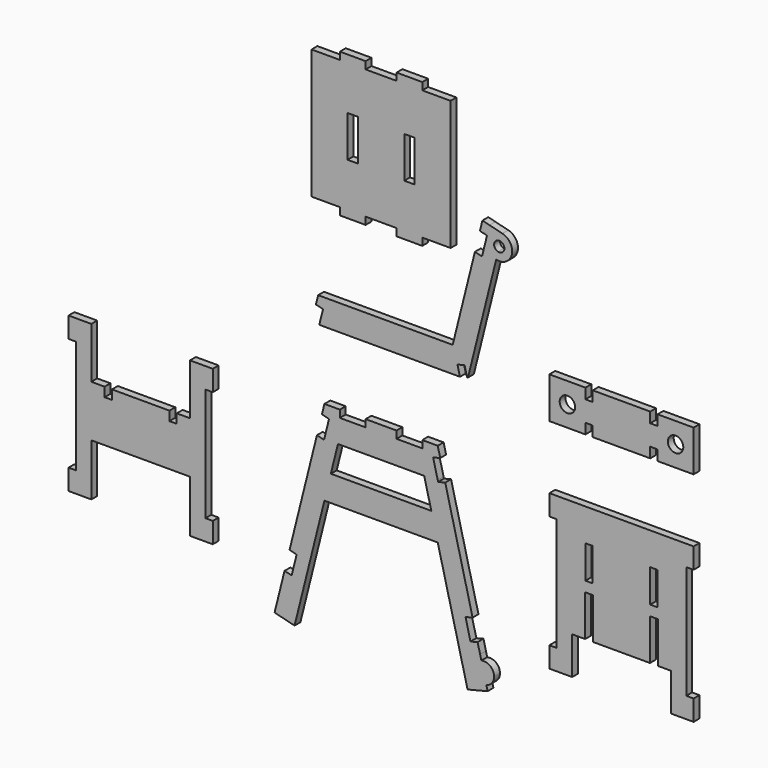
from build123d import *

# Parameters (mm, degrees)
F1_W     = 25.4
F1_H     = 101.6
F1_W_2   = 63.5
F1_H_2   = 18.034
F2_DEPTH = 18.034
F3_DEPTH = 18.034
F1_R     = 19.05
F4_DEPTH = 18.034
F1_W_3   = 18.034
F1_H_3   = 50.8
F1_H_4   = 25.4
F5_DEPTH = 18.034
F6_DEPTH = 18.034
F7_DEPTH = 18.034


# Not quite as in the source:
# - a variable given as a bare number and used for a length is read in inches; the dataset says mm whatever the document's units were


with BuildPart() as f2:
    # F1 (on Front) → F2 (new body)
    with BuildSketch(Plane.XZ):
        Polygon((91.1463229646, 1251.966), (91.1463229646, 932.434), (160.9963229646, 932.434), (224.4963229646, 932.434), (300.6963229646, 932.434), (364.1963229646, 932.434), (434.0463229646, 932.434), (434.0463229646, 1251.966), (364.1963229646, 1251.966), (300.6963229646, 1251.966), (224.4963229646, 1251.966), (160.9963229646, 1251.966), align=None)
        with Locations((192.7463229646, 1092.2)):
            Rectangle(F1_W, F1_H, mode=Mode.SUBTRACT)
        with Locations((332.4463229646, 1092.2)):
            Rectangle(F1_W, F1_H, mode=Mode.SUBTRACT)
        with Locations((332.4463229646, 1260.983)):
            Rectangle(F1_W_2, F1_H_2)
        with Locations((192.7463229646, 1260.983)):
            Rectangle(F1_W_2, F1_H_2)
        with Locations((192.7463229646, 923.417)):
            Rectangle(F1_W_2, F1_H_2)
        with Locations((332.4463229646, 923.417)):
            Rectangle(F1_W_2, F1_H_2)
    extrude(amount=F2_DEPTH)


with BuildPart() as f3:
    # F1 (on Front) → F3 (new body)
    with BuildSketch(Plane.XZ):
        with BuildLine():
            Line((143.9654091439, 723.9), (143.9654091439, 660.4))
            Line((143.9654091439, 660.4), (423.3654091439, 660.4))
            Line((423.3654091439, 660.4), (457.1344953232, 660.4))
            Line((457.1344953232, 660.4), (450.989679175, 685.0455114474))
            Line((450.989679175, 685.0455114474), (468.4879923026, 689.4083309127))
            Line((468.4879923026, 689.4083309127), (474.6328084508, 664.7628194652))
            Line((474.6328084508, 664.7628194652), (476.9525607092, 665.3411986629))
            Line((476.9525607092, 665.3411986629), (546.3859672195, 943.8233816452))
            ThreePointArc((546.3859672195, 943.8233816452), (523.2600980956, 982.3112911398), (561.7480075901, 1005.4371602637))
            Line((561.7480075901, 1005.4371602637), (529.955297823, 1013.363973095))
            Line((529.955297823, 1013.363973095), (523.8104816747, 988.7184616476))
            Line((523.8104816747, 988.7184616476), (511.5208493783, 939.4274387527))
            Line((511.5208493783, 939.4274387527), (494.0225362506, 943.790258218))
            Line((494.0225362506, 943.790258218), (439.1977373244, 723.9))
            Line((439.1977373244, 723.9), (423.3654091439, 723.9))
            Line((423.3654091439, 723.9), (143.9654091439, 723.9))
        make_face()
        Polygon((110.1963229646, 660.4), (143.9654091439, 660.4), (143.9654091439, 723.9), (107.4425649535, 723.9), (101.9152340593, 701.7310866364), (119.413547187, 697.3682671711), align=None)
        Polygon((512.4569846953, 1017.7267925602), (506.3121685471, 993.0812811128), (523.8104816747, 988.7184616476), (529.955297823, 1013.363973095), align=None)
        with BuildLine():
            ThreePointArc((561.7480075901, 1005.4371602637), (523.2600980956, 982.3112911398), (546.3859672195, 943.8233816452))
            Line((546.3859672195, 943.8233816452), (550.9945793307, 962.3075152308))
            ThreePointArc((550.9945793307, 962.3075152308), (541.7442316811, 977.7026790286), (557.139395479, 986.9530266782))
            Line((557.139395479, 986.9530266782), (561.7480075901, 1005.4371602637))
        make_face()
        with BuildLine():
            Line((550.9945793307, 962.3075152308), (546.3859672195, 943.8233816452))
            ThreePointArc((546.3859672195, 943.8233816452), (573.6142392464, 949.6109295275), (585.8169874048, 974.6302709545))
            ThreePointArc((585.8169874048, 974.6302709545), (579.0863288318, 994.1775227961), (561.7480075901, 1005.4371602637))
            Line((561.7480075901, 1005.4371602637), (557.139395479, 986.9530266782))
            ThreePointArc((557.139395479, 986.9530266782), (564.0747239756, 982.4491716911), (566.7669874048, 974.6302709545))
            ThreePointArc((566.7669874048, 974.6302709545), (561.8858881415, 964.6225343837), (550.9945793307, 962.3075152308))
        make_face()
    extrude(amount=F3_DEPTH)


with BuildPart() as f4:
    # F1 (on Front) → F4 (new body)
    with BuildSketch(Plane.XZ):
        Polygon((677.5926459293, 737.4890749257), (677.5926459293, 635.8890749257), (766.4926459293, 635.8890749257), (766.4926459293, 661.2890749257), (784.5266459293, 661.2890749257), (784.5266459293, 635.8890749257), (926.2586459293, 635.8890749257), (926.2586459293, 661.2890749257), (944.2926459293, 661.2890749257), (944.2926459293, 635.8890749257), (1033.1926459293, 635.8890749257), (1033.1926459293, 737.4890749257), (944.2926459293, 737.4890749257), (944.2926459293, 712.0890749257), (926.2586459293, 712.0890749257), (926.2586459293, 737.4890749257), (784.5266459293, 737.4890749257), (784.5266459293, 712.0890749257), (766.4926459293, 712.0890749257), (766.4926459293, 737.4890749257), align=None)
        with Locations((722.0426459293, 686.6890749257)):
            Circle(F1_R, mode=Mode.SUBTRACT)
        with Locations((988.7426459293, 686.6890749257)):
            Circle(F1_R, mode=Mode.SUBTRACT)
    extrude(amount=F4_DEPTH)


with BuildPart() as f5:
    # F1 (on Front) → F5 (new body)
    with BuildSketch(Plane.XZ):
        with Locations((686.6096459293, 454.1820457896)):
            Rectangle(F1_W_3, F1_H_3)
        Polygon((695.6266459293, 149.3820457896), (695.6266459293, 98.5820457896), (733.7266459293, 98.5820457896), (733.7266459293, 191.4648930249), (733.7266459293, 479.5820457896), (695.6266459293, 479.5820457896), (695.6266459293, 428.7820457896), align=None)
        with Locations((686.6096459293, 123.9820457896)):
            Rectangle(F1_W_3, F1_H_3)
        Polygon((733.7266459293, 479.5820457896), (733.7266459293, 191.4648930249), (765.8576459293, 191.4648930249), (765.8576459293, 293.0648930249), (766.4926459293, 293.0648930249), (766.4926459293, 318.4648930249), (766.4926459293, 399.7448930249), (784.5266459293, 399.7448930249), (784.5266459293, 318.4648930249), (784.5266459293, 293.0648930249), (785.1616459293, 293.0648930249), (785.1616459293, 191.4648930249), (855.3926459293, 191.4648930249), (925.6236459293, 191.4648930249), (925.6236459293, 293.0648930249), (926.2586459293, 293.0648930249), (926.2586459293, 318.4648930249), (926.2586459293, 399.7448930249), (944.2926459293, 399.7448930249), (944.2926459293, 318.4648930249), (944.2926459293, 293.0648930249), (944.9276459293, 293.0648930249), (944.9276459293, 191.4648930249), (977.0586459293, 191.4648930249), (977.0586459293, 479.5820457896), align=None)
        with Locations((775.5096459293, 305.7648930249)):
            Rectangle(F1_W_3, F1_H_4)
        with Locations((935.2756459293, 305.7648930249)):
            Rectangle(F1_W_3, F1_H_4)
        Polygon((977.0586459293, 191.4648930249), (977.0586459293, 98.5820457896), (1015.1586459293, 98.5820457896), (1015.1586459293, 149.3820457896), (1015.1586459293, 428.7820457896), (1015.1586459293, 479.5820457896), (977.0586459293, 479.5820457896), align=None)
        with Locations((1024.1756459293, 454.1820457896)):
            Rectangle(F1_W_3, F1_H_3)
        with Locations((1024.1756459293, 123.9820457896)):
            Rectangle(F1_W_3, F1_H_3)
    extrude(amount=F5_DEPTH)


with BuildPart() as f6:
    # F1 (on Front) → F6 (new body)
    with BuildSketch(Plane.XZ):
        Polygon((122.8963229646, 416.7102289482), (156.252701519, 416.7102289482), (170.7551141323, 474.8762289482), (160.9963229646, 474.8762289482), (160.9963229646, 483.4108320399), (122.8963229646, 492.9102289482), (122.8963229646, 466.7326427627), (134.2498199441, 463.9018980356), (122.8963229646, 418.3655088215), align=None)
        Polygon((122.8963229646, 492.9102289482), (116.7515068164, 468.2647175008), (122.8963229646, 466.7326427627), align=None)
        Polygon((160.9963229646, 492.9102289482), (122.8963229646, 492.9102289482), (160.9963229646, 483.4108320399), align=None)
        Polygon((364.1963229646, 492.9102289482), (364.1963229646, 483.4108320399), (402.2963229646, 492.9102289482), align=None)
        Polygon((354.4375317969, 474.8762289482), (368.9399444103, 416.7102289482), (402.2963229646, 416.7102289482), (402.2963229646, 418.3655088215), (390.9428259852, 463.9018980356), (402.2963229646, 466.7326427627), (402.2963229646, 492.9102289482), (364.1963229646, 483.4108320399), (364.1963229646, 474.8762289482), align=None)
        Polygon((170.7551141323, 474.8762289482), (156.252701519, 416.7102289482), (368.9399444103, 416.7102289482), (354.4375317969, 474.8762289482), (300.6963229646, 474.8762289482), (300.6963229646, 492.9102289482), (224.4963229646, 492.9102289482), (224.4963229646, 474.8762289482), align=None)
        Polygon((24.5792645929, 98.5820457896), (0, 0), (49.2910228948, -12.2896322965), (122.8963229646, 282.9251018307), (122.8963229646, 346.4251018307), (138.7286511452, 346.4251018307), (156.252701519, 416.7102289482), (122.8963229646, 416.7102289482), (122.8963229646, 418.3655088215), (121.9601876476, 414.6108751407), (104.4618745199, 418.973694606), (36.8688968894, 147.8730686845), (54.3672100171, 143.5102492192), (42.0775777206, 94.2192263244), align=None)
        Polygon((122.8963229646, 346.4251018307), (122.8963229646, 282.9251018307), (138.7286511452, 346.4251018307), align=None)
        Polygon((138.7286511452, 346.4251018307), (122.8963229646, 282.9251018307), (402.2963229646, 282.9251018307), (386.4639947841, 346.4251018307), align=None)
        Polygon((386.4639947841, 346.4251018307), (402.2963229646, 282.9251018307), (402.2963229646, 346.4251018307), align=None)
        with BuildLine():
            Line((402.2963229646, 346.4251018307), (402.2963229646, 282.9251018307))
            Line((402.2963229646, 282.9251018307), (475.9016230344, -12.2896322965))
            Line((475.9016230344, -12.2896322965), (525.1926459293, 0))
            ThreePointArc((525.1926459293, 0), (479.0071545358, 27.7510429488), (506.7581974846, 73.9365343422))
            Line((506.7581974846, 73.9365343422), (500.6133813363, 98.5820457896))
            Line((500.6133813363, 98.5820457896), (483.1150682087, 94.2192263244))
            Line((483.1150682087, 94.2192263244), (470.8254359122, 143.5102492192))
            Line((470.8254359122, 143.5102492192), (488.3237490399, 147.8730686845))
            Line((488.3237490399, 147.8730686845), (427.755494449, 390.7990693751))
            Line((427.755494449, 390.7990693751), (420.7307714093, 418.973694606))
            Line((420.7307714093, 418.973694606), (403.2324582817, 414.6108751407))
            Line((403.2324582817, 414.6108751407), (402.2963229646, 418.3655088215))
            Line((402.2963229646, 418.3655088215), (402.2963229646, 416.7102289482))
            Line((402.2963229646, 416.7102289482), (368.9399444103, 416.7102289482))
            Line((368.9399444103, 416.7102289482), (386.4639947841, 346.4251018307))
            Line((386.4639947841, 346.4251018307), (402.2963229646, 346.4251018307))
        make_face()
        with BuildLine():
            ThreePointArc((509.8306055587, 61.6137786185), (491.3299102595, 30.8234510229), (522.1202378551, 12.3227557237))
            Line((522.1202378551, 12.3227557237), (509.8306055587, 61.6137786185))
        make_face()
        with BuildLine():
            ThreePointArc((506.7581974846, 73.9365343422), (479.0071545358, 27.7510429488), (525.1926459293, 0))
            Line((525.1926459293, 0), (522.1202378551, 12.3227557237))
            ThreePointArc((522.1202378551, 12.3227557237), (491.3299102595, 30.8234510229), (509.8306055587, 61.6137786185))
            Line((509.8306055587, 61.6137786185), (506.7581974846, 73.9365343422))
        make_face()
        with BuildLine():
            Line((509.8306055587, 61.6137786185), (522.1202378551, 12.3227557237))
            ThreePointArc((522.1202378551, 12.3227557237), (535.9908948485, 21.3304656978), (541.3754217069, 36.9682671711))
            ThreePointArc((541.3754217069, 36.9682671711), (531.6132231802, 56.9837403127), (509.8306055587, 61.6137786185))
        make_face()
        Polygon((402.2963229646, 492.9102289482), (402.2963229646, 466.7326427627), (408.4411391129, 468.2647175008), align=None)
    extrude(amount=F6_DEPTH)


with BuildPart() as f7:
    # F1 (on Front) → F7 (new body)
    with BuildSketch(Plane.XZ):
        with Locations((-498.983, 454.1820457896)):
            Rectangle(F1_W_3, F1_H_3)
        Polygon((-489.966, 98.5820457896), (-451.866, 98.5820457896), (-451.866, 227.0124772853), (-451.866, 354.0124772853), (-451.866, 479.5820457896), (-489.966, 479.5820457896), (-489.966, 428.7820457896), (-489.966, 149.3820457896), align=None)
        with Locations((-498.983, 123.9820457896)):
            Rectangle(F1_W_3, F1_H_3)
        Polygon((-451.866, 354.0124772853), (-451.866, 227.0124772853), (-330.2, 227.0124772853), (-330.2, 354.0124772853), (-401.066, 354.0124772853), (-401.066, 331.1648930249), (-419.1, 331.1648930249), (-419.1, 354.0124772853), align=None)
        Polygon((-330.2, 227.0124772853), (-208.534, 227.0124772853), (-208.534, 354.0124772853), (-241.3, 354.0124772853), (-241.3, 331.1648930249), (-259.334, 331.1648930249), (-259.334, 354.0124772853), (-330.2, 354.0124772853), align=None)
        Polygon((-208.534, 98.5820457896), (-170.434, 98.5820457896), (-170.434, 149.3820457896), (-170.434, 428.7820457896), (-170.434, 479.5820457896), (-208.534, 479.5820457896), (-208.534, 354.0124772853), (-208.534, 227.0124772853), align=None)
        with Locations((-161.417, 454.1820457896)):
            Rectangle(F1_W_3, F1_H_3)
        with Locations((-161.417, 123.9820457896)):
            Rectangle(F1_W_3, F1_H_3)
    extrude(amount=F7_DEPTH)


solid = Compound([f2.part, f3.part, f4.part, f5.part, f6.part, f7.part])
